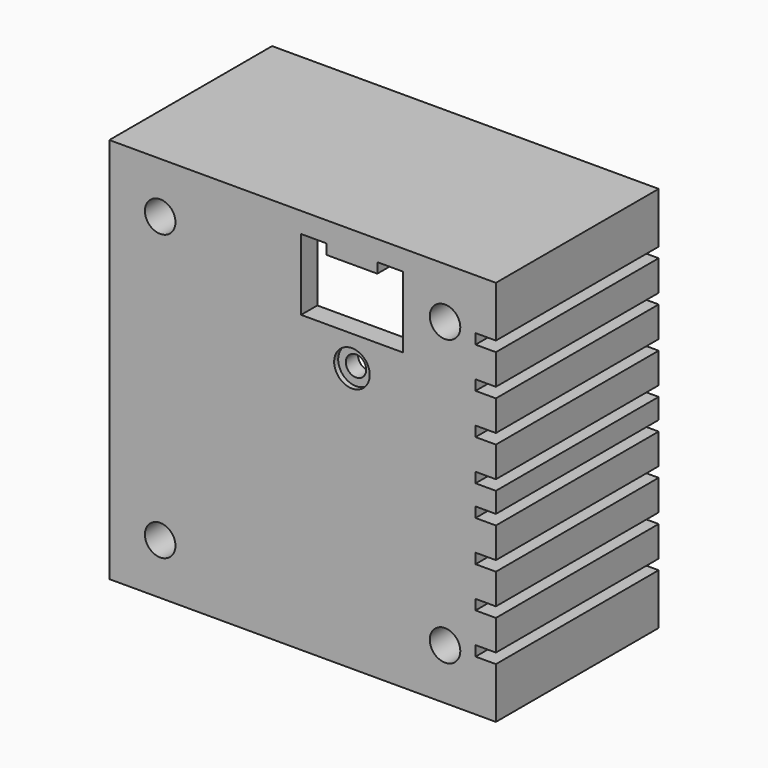
from build123d import *

# Parameters (mm, degrees)
F0_W      = 2
F0_H      = 2
F1_DEPTH  = 3
F0_H_2    = 14
F0_W_2    = 14
F0_W_3    = 11
F2_DEPTH  = 2
F0_R      = 2.5
F3_DEPTH  = 4
F0_R_2    = 1.5
F0_R_3    = 0.95
F4_DEPTH  = 20
F5_DEPTH  = 17
F6_DEPTH  = 17
F7_DEPTH  = 17
F8_DEPTH  = 17
F0_W_4    = 6
F0_H_3    = 6
F9_DEPTH  = 2
F0_H_4    = 3
F10_DEPTH = 20
F0_W_5    = 3
F0_W_6    = 5
F0_W_7    = 1.1521804929
F0_H_5    = 5
F0_R_4    = 1.75
F0_R_5    = 1
F0_W_8    = 0.8478195071
F11_DEPTH = 2
F0_H_6    = 1
F12_DEPTH = 4
F0_W_9    = 2.5
F13_DEPTH = 4
F14_DEPTH = 2
F15_DEPTH = 2
F16_DEPTH = 0.5


# Not quite as in the source:
# - a feature names something its author has since deleted; it is built from what else it names


with BuildPart() as f1:
    # F0 (on Front) → F1 (new body)
    with BuildSketch(Plane.XZ):
        Polygon((16, 1), (16, 2), (2, 2), (1, 2), (-1, 2), (-1, 10), (-1, 16), (-2, 16), (-2, 2), (-4, 2), (-4, 16), (-5, 16), (-5, 2), (-16, 2), (-16, 1), (-5, 1), (-5, -1), (-16, -1), (-16, -2), (-5, -2), (-5, -16), (-4, -16), (-4, -2), (-2, -2), (-2, -16), (-1, -16), (-1, -2), (1, -2), (1, -16), (2, -16), (2, -2), (16, -2), (16, -1), (2, -1), (2, 1), align=None)
        with Locations((-3, 0)):
            Rectangle(F0_W, F0_H, mode=Mode.SUBTRACT)
        Rectangle(F0_W, F0_H, mode=Mode.SUBTRACT)
    extrude(amount=-F1_DEPTH)

    # F0 (on Front) → F2 (join)
    with BuildSketch(Plane.XZ):
        Polygon((16, 2), (16, 10.1685791543), (16, 11), (11, 11), (9.8478195071, 11), (9.8478195071, 10.2023985237), (9.8478195071, 10), (7.6956390142, 10), (7.6956390142, 7.9433578615), (7.6956390142, 6.0566421385), (7.6956390142, 4), (4.8478195071, 4), (2, 4), (2, 6.0566421385), (2, 7.9433578615), (2, 10), (-0.1521804929, 10), (-1, 10), (-1, 2), (1, 2), (2, 2), align=None)
        with Locations((-3, 9)):
            Rectangle(F0_W, F0_H_2)
        Polygon((16, -11), (16, -2), (2, -2), (2, -16), (11, -16), (11, -11), align=None)
        with Locations((9, 0)):
            Rectangle(F0_W_2, F0_H)
        with Locations((-10.5, 0)):
            Rectangle(F0_W_3, F0_H)
        Polygon((-11, -11), (-11, -16), (-5, -16), (-5, -2), (-16, -2), (-16, -11), align=None)
        with Locations((-3, -9)):
            Rectangle(F0_W, F0_H_2)
        with Locations((0, -9)):
            Rectangle(F0_W, F0_H_2)
        Polygon((-5, 2), (-5, 16), (-11, 16), (-11, 11), (-16, 11), (-16, 10), (-10, 10), (-10, 4), (-16, 4), (-16, 2), align=None)
        with Locations((-3, 0)):
            Rectangle(F0_W, F0_H)
        Rectangle(F0_W, F0_H)
    extrude(amount=-F2_DEPTH)

    # F0 (on Front) → F3 (join)
    with BuildSketch(Plane.XZ):
        Polygon((11, 11), (16, 11), (17, 11), (17, 13), (17, 14), (17, 17), (14, 17), (11, 17), (11, 16), align=None)
        with Locations((14, 14)):
            Circle(F0_R, mode=Mode.SUBTRACT)
        Polygon((-11, 16), (-11, 17), (-14, 17), (-17, 17), (-17, 14), (-17, 11), (-16, 11), (-11, 11), align=None)
        with Locations((-14, 14)):
            Circle(F0_R, mode=Mode.SUBTRACT)
        Polygon((-14, -17), (-11, -17), (-11, -16), (-11, -11), (-16, -11), (-17, -11), (-17, -14), (-17, -17), align=None)
        with Locations((-14, -14)):
            Circle(F0_R, mode=Mode.SUBTRACT)
        Polygon((17, -11), (16, -11), (11, -11), (11, -16), (11, -17), (14, -17), (17, -17), (17, -14), (17, -13), align=None)
        with Locations((14, -14)):
            Circle(F0_R, mode=Mode.SUBTRACT)
    extrude(amount=-F3_DEPTH)

    # F0 (on Front) → F4 (join)
    with BuildSketch(Plane.XZ):
        with Locations((14, 14)):
            Circle(F0_R)
        with Locations((14, 14)):
            Circle(F0_R_2, mode=Mode.SUBTRACT)
        with Locations((14, 14)):
            Circle(F0_R_2)
        with Locations((14, 14)):
            Circle(F0_R_3, mode=Mode.SUBTRACT)
        with Locations((-14, 14)):
            Circle(F0_R)
        with Locations((-14, 14)):
            Circle(F0_R_2, mode=Mode.SUBTRACT)
        with Locations((-14, 14)):
            Circle(F0_R_2)
        with Locations((-14, 14)):
            Circle(F0_R_3, mode=Mode.SUBTRACT)
        with Locations((-14, -14)):
            Circle(F0_R)
        with Locations((-14, -14)):
            Circle(F0_R_2, mode=Mode.SUBTRACT)
        with Locations((-14, -14)):
            Circle(F0_R_2)
        with Locations((-14, -14)):
            Circle(F0_R_3, mode=Mode.SUBTRACT)
        with Locations((14, -14)):
            Circle(F0_R)
        with Locations((14, -14)):
            Circle(F0_R_2, mode=Mode.SUBTRACT)
        with Locations((14, -14)):
            Circle(F0_R_2)
        with Locations((14, -14)):
            Circle(F0_R_3, mode=Mode.SUBTRACT)
    extrude(amount=-F4_DEPTH)

    # F0 (on Front) → F5 (cut)
    with BuildSketch(Plane.XZ):
        with Locations((-14, 14)):
            Circle(F0_R_2)
        with Locations((-14, 14)):
            Circle(F0_R_3, mode=Mode.SUBTRACT)
    extrude(amount=-F5_DEPTH, mode=Mode.SUBTRACT)

    # F0 (on Front) → F6 (cut)
    with BuildSketch(Plane.XZ):
        with Locations((14, 14)):
            Circle(F0_R_2)
        with Locations((14, 14)):
            Circle(F0_R_3, mode=Mode.SUBTRACT)
    extrude(amount=-F6_DEPTH, mode=Mode.SUBTRACT)

    # F0 (on Front) → F7 (cut)
    with BuildSketch(Plane.XZ):
        with Locations((-14, -14)):
            Circle(F0_R_2)
        with Locations((-14, -14)):
            Circle(F0_R_3, mode=Mode.SUBTRACT)
    extrude(amount=-F7_DEPTH, mode=Mode.SUBTRACT)

    # F0 (on Front) → F8 (cut)
    with BuildSketch(Plane.XZ):
        with Locations((14, -14)):
            Circle(F0_R_2)
        with Locations((14, -14)):
            Circle(F0_R_3, mode=Mode.SUBTRACT)
    extrude(amount=-F8_DEPTH, mode=Mode.SUBTRACT)

    # F0 (on Front) → F9 (join)
    with BuildSketch(Plane.XZ):
        with Locations((-13, 7)):
            Rectangle(F0_W_4, F0_H_3)
    extrude(amount=-F9_DEPTH)

    # F0 (on Front) → F10, piece 6 (join)
    with BuildSketch(Plane.XZ):
        with Locations((18, 18)):
            Rectangle(F0_W, F0_H)
        with Locations((18, 15.5)):
            Rectangle(F0_W, F0_H_4)
        with Locations((15.5, 18)):
            Rectangle(F0_W_5, F0_H)
        Polygon((9.8478195071, 17), (11, 17), (14, 17), (14, 19), (7.3478195071, 19), (7.3478195071, 17), align=None)
        with Locations((4.8478195071, 18)):
            Rectangle(F0_W_6, F0_H)
        Polygon((-0.1521804929, 17), (2.3478195071, 17), (2.3478195071, 19), (-14, 19), (-14, 17), (-11, 17), align=None)
        with Locations((-15.5, 18)):
            Rectangle(F0_W_5, F0_H)
        with Locations((-18, 18)):
            Rectangle(F0_W, F0_H)
        with Locations((-18, 15.5)):
            Rectangle(F0_W, F0_H_4)
        Polygon((-19, -14), (-17, -14), (-17, -11), (-17, -2), (-17, -1), (-17, 1), (-17, 2), (-17, 11), (-17, 14), (-19, 14), align=None)
        Polygon((17, 13), (17, 11), (17, 10), (19, 10), (19, 13), align=None)
        Polygon((17, -10), (17, -11), (17, -13), (19, -13), (19, -10), align=None)
        with Locations((18, -15.5)):
            Rectangle(F0_W, F0_H_4)
        with Locations((18, -18)):
            Rectangle(F0_W, F0_H)
        with Locations((15.5, -18)):
            Rectangle(F0_W_5, F0_H)
        Polygon((14, -17), (11, -17), (-11, -17), (-14, -17), (-14, -19), (14, -19), align=None)
        with Locations((-15.5, -18)):
            Rectangle(F0_W_5, F0_H)
        with Locations((-18, -18)):
            Rectangle(F0_W, F0_H)
        with Locations((-18, -15.5)):
            Rectangle(F0_W, F0_H_4)
    extrude(amount=-F10_DEPTH)

    # F0 (on Front) → F11 (join)
    with BuildSketch(Plane.XZ):
        with Locations((10.4239097536, 13.5)):
            Rectangle(F0_W_7, F0_H_5)
        with BuildLine():
            Line((7.6956390142, 7.9433578615), (7.6956390142, 10))
            Line((7.6956390142, 10), (4.8478195071, 10))
            ThreePointArc((4.8478195071, 10), (6.6042258404, 9.4320848653), (7.6956390142, 7.9433578615))
        make_face()
        with BuildLine():
            ThreePointArc((7.6956390142, 7.9433578615), (6.6042258404, 9.4320848653), (4.8478195071, 10))
            ThreePointArc((4.8478195071, 10), (3.0914131738, 9.4320848653), (2, 7.9433578615))
            Line((2, 7.9433578615), (2, 6.0566421385))
            ThreePointArc((2, 6.0566421385), (3.0914131738, 4.5679151347), (4.8478195071, 4))
            ThreePointArc((4.8478195071, 4), (6.6042258404, 4.5679151347), (7.6956390142, 6.0566421385))
            Line((7.6956390142, 6.0566421385), (7.6956390142, 7.9433578615))
        make_face()
        with Locations((4.8478195071, 7)):
            Circle(F0_R_4, mode=Mode.SUBTRACT)
        with BuildLine():
            Line((7.6956390142, 4), (7.6956390142, 6.0566421385))
            ThreePointArc((7.6956390142, 6.0566421385), (6.6042258404, 4.5679151347), (4.8478195071, 4))
            Line((4.8478195071, 4), (7.6956390142, 4))
        make_face()
        with Locations((4.8478195071, 7)):
            Circle(F0_R_4)
        with Locations((4.8478195071, 7)):
            Circle(F0_R_5, mode=Mode.SUBTRACT)
        with BuildLine():
            ThreePointArc((4.8478195071, 4), (3.0914131738, 4.5679151347), (2, 6.0566421385))
            Line((2, 6.0566421385), (2, 4))
            Line((2, 4), (4.8478195071, 4))
        make_face()
        with BuildLine():
            Line((4.8478195071, 10), (2, 10))
            Line((2, 10), (2, 7.9433578615))
            ThreePointArc((2, 7.9433578615), (3.0914131738, 9.4320848653), (4.8478195071, 10))
        make_face()
        with Locations((-0.5760902464, 13)):
            Rectangle(F0_W_8, F0_H_3)
    extrude(amount=-F11_DEPTH)



with BuildPart() as f10:
    # F0 (on Front) → F10 (new body)
    with BuildSketch(Plane.XZ):
        with Locations((18, 7.5)):
            Rectangle(F0_W, F0_H_4)
    extrude(amount=-F10_DEPTH)


with BuildPart() as f10b:
    # F0 (on Front) → F10, piece 2 (new body)
    with BuildSketch(Plane.XZ):
        with Locations((18, 3.5)):
            Rectangle(F0_W, F0_H_4)
    extrude(amount=-F10_DEPTH)


with BuildPart() as f10c:
    # F0 (on Front) → F10, piece 3 (new body)
    with BuildSketch(Plane.XZ):
        Polygon((19, 1), (17, 1), (17, 0), (17, -1), (19, -1), (19, 0), align=None)
    extrude(amount=-F10_DEPTH)


with BuildPart() as f10d:
    # F0 (on Front) → F10, piece 4 (new body)
    with BuildSketch(Plane.XZ):
        with Locations((18, -3.5)):
            Rectangle(F0_W, F0_H_4)
    extrude(amount=-F10_DEPTH)


with BuildPart() as f10e:
    # F0 (on Front) → F10, piece 5 (new body)
    with BuildSketch(Plane.XZ):
        with Locations((18, -7.5)):
            Rectangle(F0_W, F0_H_4)
    extrude(amount=-F10_DEPTH)


with BuildPart() as f1_1:
    add(f1.part)

    add(f10.part)  # F12 merges F10

    add(f10b.part)  # F12 merges F10b

    add(f10c.part)  # F12 merges F10c

    add(f10d.part)  # F12 merges F10d

    add(f10e.part)  # F12 merges F10e
    # F0 (on Front) → F12 (join)
    with BuildSketch(Plane.XZ):
        Polygon((16, 11), (16, 10.1685791543), (16, 2), (16, 1), (16, -1), (16, -2), (16, -11), (17, -11), (17, -10), (17, -9), (17, -6), (17, -5), (17, -2), (17, -1), (17, 0), (17, 1), (17, 2), (17, 5), (17, 6), (17, 9), (17, 10), (17, 11), align=None)
        with Locations((4.8478195071, 16.5)):
            Rectangle(F0_W_6, F0_H_6)
        Polygon((11, -16), (2, -16), (1, -16), (-1, -16), (-2, -16), (-4, -16), (-5, -16), (-11, -16), (-11, -17), (11, -17), align=None)
        Polygon((-2, 16), (-1, 16), (-0.1521804929, 16), (-0.1521804929, 17), (-11, 17), (-11, 16), (-5, 16), (-4, 16), align=None)
        Polygon((-16, 1), (-16, 2), (-16, 4), (-16, 10), (-16, 11), (-17, 11), (-17, 2), (-17, 1), (-17, -1), (-17, -2), (-17, -11), (-16, -11), (-16, -2), (-16, -1), align=None)
    extrude(amount=-F12_DEPTH)

    # F0 (on Front) → F13 (join)
    with BuildSketch(Plane.XZ):
        with Locations((10.4239097536, 16.5)):
            Rectangle(F0_W_7, F0_H_6)
        with Locations((8.5978195071, 16.5)):
            Rectangle(F0_W_9, F0_H_6)
        Polygon((2, 16), (2.3478195071, 16), (2.3478195071, 17), (-0.1521804929, 17), (-0.1521804929, 16), (1, 16), align=None)
    extrude(amount=-F13_DEPTH)

    # F0 (on Front) → F14 (cut)
    with BuildSketch(Plane.XZ):
        Polygon((2, 16), (2.3478195071, 16), (2.3478195071, 17), (-0.1521804929, 17), (-0.1521804929, 16), (1, 16), align=None)
    extrude(amount=-F14_DEPTH, mode=Mode.SUBTRACT)

    # F0 (on Front) → F15 (cut)
    with BuildSketch(Plane.XZ):
        with Locations((8.5978195071, 16.5)):
            Rectangle(F0_W_9, F0_H_6)
    extrude(amount=-F15_DEPTH, mode=Mode.SUBTRACT)

    # F0 (on Front) → F16 (cut)
    with BuildSketch(Plane.XZ):
        with Locations((4.8478195071, 7)):
            Circle(F0_R_4)
        with Locations((4.8478195071, 7)):
            Circle(F0_R_5, mode=Mode.SUBTRACT)
    extrude(amount=-F16_DEPTH, mode=Mode.SUBTRACT)


solid = f1_1.part
